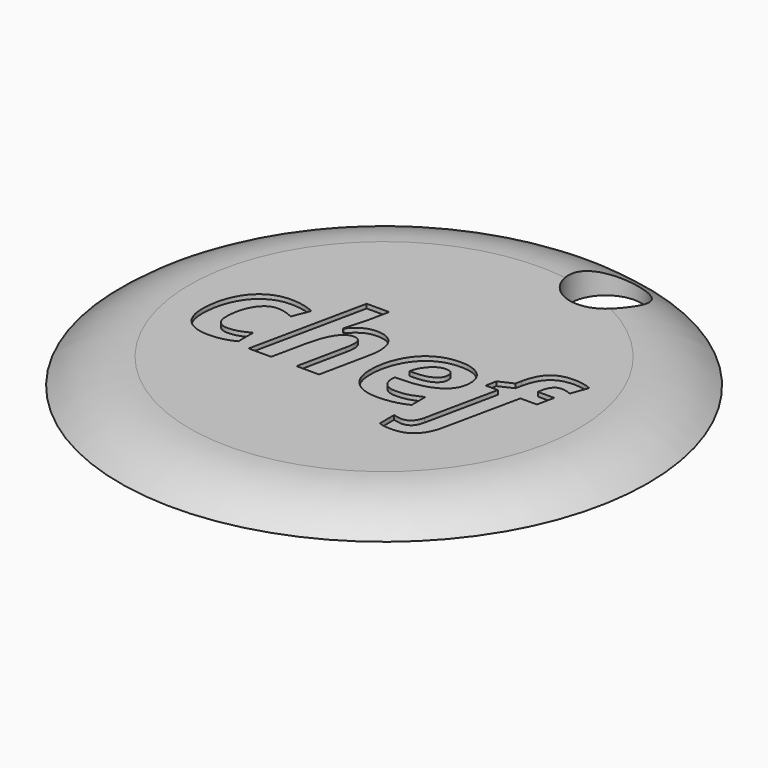
from build123d import *

# Parameters (mm, degrees)
F0_R         = 62.7695987609
F1_DEPTH     = 6.096
F2_R         = 8.559644156
F5_DEPTH     = 6.097
F7_TEXT_SIZE = 36.514049351
F8_DEPTH     = 1


# Not quite as in the source:
# - a fillet or chamfer that OpenCascade refuses, or shapes differently, is made with other operations: its cross-section is extruded or revolved along the edge and cut away or added
# - the program builds the solid bodies; features that only make, move or delete a surface that nothing else refers to are left out
# - Text() gives the source's letters only with a copy of the font that has no kerning and outlines rounded to 1/6400 em; it was checked with that copy


with BuildPart() as f1:
    # F0 (on Top) → F1 (new body)
    with BuildSketch(Plane.XY):
        Circle(F0_R)
    extrude(amount=F1_DEPTH)

    # F2 (on face) → F5 (cut, through all)
    with BuildSketch(Plane.XY.offset(6.096)):
        with Locations((14.7785907611, 47.4341027439)):
            Circle(F2_R)
    extrude(amount=-F5_DEPTH, mode=Mode.SUBTRACT)

    # F6: fillet of radius 25.4 on 1 edges, made by hand

    # F6_s1 → F6_t2 (revolve, cut)
    with BuildSketch(Plane.XZ):
        with BuildLine():
            ThreePointArc((62.7695987609, 0), (55.0603708251, 4.5233120599), (46.2615527226, 6.096))
            Line((46.2615527226, 6.096), (62.7695987609, 6.096))
            Line((62.7695987609, 6.096), (62.7695987609, 0))
        make_face()
    revolve(axis=Axis((0, 0, 6.096), (0, 0, 1)), mode=Mode.SUBTRACT)

    # F7 (on face) → F8 (cut)
    with BuildSketch(Plane.XY.offset(6.096)):
        with Locations((-40, -13.1450577664)):
            Text('chef', F7_TEXT_SIZE, font='Open Sans', font_style=FontStyle.BOLDITALIC, text_align=(TextAlign.LEFT, TextAlign.BOTTOM))
    extrude(amount=-F8_DEPTH, mode=Mode.SUBTRACT)


solid = f1.part
